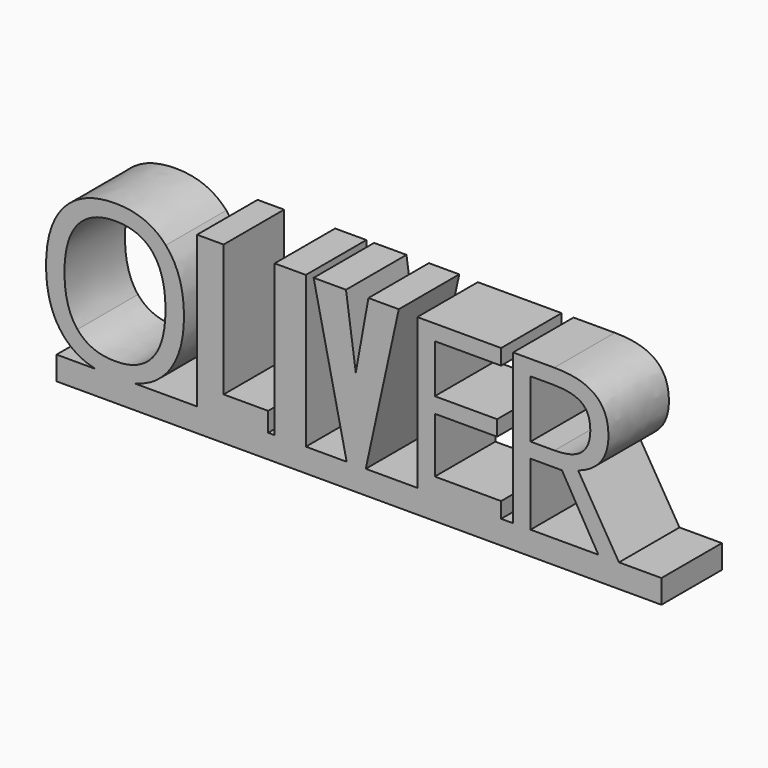
from build123d import *

# Parameters (mm, degrees)
F0_W         = 10.3234383059
F0_H         = 50
F0_TEXT_SIZE = 69.6380393088
F1_DEPTH     = 25


# Not quite as in the source:
# - Text() gives the source's letters only with a copy of the font that has no kerning and outlines rounded to 1/6400 em; it was checked with that copy


with BuildPart() as f1:
    # F0 (on Front) → F1 (new body)
    with BuildSketch(Plane.XZ):
        Polygon((-25.6522880155, 16.8570160866), (-25.6522880155, -33.1429839134), (-16.8708102065, -33.1429839134), (-2.1405949011, -33.1429839134), (-2.1405949011, -26.771583315), (-16.8708102065, -26.771583315), (-16.8708102065, 16.8570160866), align=None)
        with BuildLine():
            Line((-16.8708102065, -33.1429839134), (-25.6522880155, -33.1429839134))
            Line((-25.6522880155, -33.1429839134), (-46.4257544633, -33.1429839134))
            add(Edge.make_bspline(
                [(-46.4257544633, -33.1429839134), (-49.3466087915, -33.8265776634), (-52.7373318548, -33.8265776634)],
                knots=[0.6833950988, 0.6833950988, 0.6833950988, 1, 1, 1], degree=2))
            add(Edge.make_bspline(
                [(-52.7373318548, -33.8265776634), (-56.2343710014, -33.8265776634), (-59.2216208008, -33.1429839134)],
                knots=[0, 0, 0, 0.319412416, 0.319412416, 0.319412416], degree=2))
            Line((-59.2216208008, -33.1429839134), (-72.1091241795, -33.1429839134))
            Line((-72.1091241795, -33.1429839134), (-72.1091241795, -40.935254842))
            Line((-72.1091241795, -40.935254842), (127.8908758205, -40.935254842))
            Line((127.8908758205, -40.935254842), (127.8908758205, -33.1429839134))
            Line((127.8908758205, -33.1429839134), (113.8607155293, -33.1429839134))
            Line((113.8607155293, -33.1429839134), (107.0274829221, -33.1429839134))
            Line((107.0274829221, -33.1429839134), (84.6127390196, -33.1429839134))
            Line((84.6127390196, -33.1429839134), (78.8349579457, -33.1429839134))
            Line((78.8349579457, -33.1429839134), (74.8870150825, -33.1429839134))
            Line((74.8870150825, -33.1429839134), (47.1732516263, -33.1429839134))
            Line((47.1732516263, -33.1429839134), (30.120832633, -33.1429839134))
            Line((30.120832633, -33.1429839134), (23.8147727107, -33.1429839134))
            Line((23.8147727107, -33.1429839134), (10.3234383059, -33.1429839134))
            Line((10.3234383059, -33.1429839134), (0, -33.1429839134))
            Line((0, -33.1429839134), (-2.1405949011, -33.1429839134))
            Line((-2.1405949011, -33.1429839134), (-16.8708102065, -33.1429839134))
        make_face()
        with BuildLine():
            add(Edge.make_bspline(
                [(-46.4257544633, -33.1429839134), (-49.3466087915, -33.8265776634), (-52.7373318548, -33.8265776634)],
                knots=[0.6833950988, 0.6833950988, 0.6833950988, 1, 1, 1], degree=2))
            Line((-46.4257544633, -33.1429839134), (-59.2216208008, -33.1429839134))
            add(Edge.make_bspline(
                [(-52.7373318548, -33.8265776634), (-56.2343710014, -33.8265776634), (-59.2216208008, -33.1429839134)],
                knots=[0, 0, 0, 0.319412416, 0.319412416, 0.319412416], degree=2))
        make_face()
        with BuildLine():
            Line((-59.2216208008, -33.1429839134), (-46.4257544633, -33.1429839134))
            add(Edge.make_bspline(
                [(-36.0055610215, -27.0069162051), (-40.1210588494, -31.667439421), (-46.4257544633, -33.1429839134)],
                knots=[0, 0, 0, 0.6833950988, 0.6833950988, 0.6833950988], degree=2))
            add(Edge.make_bspline(
                [(-29.9834256048, -8.2840429412), (-29.9834256048, -20.1872547468), (-36.0055610215, -27.0069162051)],
                knots=[0, 0, 0, 1, 1, 1], degree=2))
            add(Edge.make_bspline(
                [(-35.9838596326, 10.4334049755), (-29.9834256048, 3.6517209477), (-29.9834256048, -8.2840429412)],
                knots=[0, 0, 0, 1, 1, 1], degree=2))
            add(Edge.make_bspline(
                [(-52.6722276882, 17.2150890032), (-41.9842936604, 17.2150890032), (-35.9838596326, 10.4334049755)],
                knots=[0, 0, 0, 1, 1, 1], degree=2))
            add(Edge.make_bspline(
                [(-69.6210124104, 10.5527626144), (-63.653130466, 17.2150890032), (-52.6722276882, 17.2150890032)],
                knots=[0, 0, 0, 1, 1, 1], degree=2))
            add(Edge.make_bspline(
                [(-75.5888943548, -8.2189387745), (-75.5888943548, 3.8904362255), (-69.6210124104, 10.5527626144)],
                knots=[0, 0, 0, 1, 1, 1], degree=2))
            add(Edge.make_bspline(
                [(-69.6372884521, -27.126273844), (-75.5888943548, -20.4259700245), (-75.5888943548, -8.2189387745)],
                knots=[0, 0, 0, 1, 1, 1], degree=2))
            add(Edge.make_bspline(
                [(-59.2216208008, -33.1429839134), (-65.5866993698, -31.6864174325), (-69.6372884521, -27.126273844)],
                knots=[0.319412416, 0.319412416, 0.319412416, 1, 1, 1], degree=2))
        make_face()
        with BuildLine():
            add(Edge.make_bspline(
                [(-69.4908040771, -8.2840429412), (-69.4908040771, -18.3534873856), (-65.1993544243, -23.561820719)],
                knots=[0, 0, 0, 1, 1, 1], degree=2))
            add(Edge.make_bspline(
                [(-65.1993544243, 6.8526758088), (-69.4908040771, 1.6443424755), (-69.4908040771, -8.2840429412)],
                knots=[0, 0, 0, 1, 1, 1], degree=2))
            add(Edge.make_bspline(
                [(-52.6722276882, 12.0610091421), (-60.9079047715, 12.0610091421), (-65.1993544243, 6.8526758088)],
                knots=[0, 0, 0, 1, 1, 1], degree=2))
            add(Edge.make_bspline(
                [(-40.2807346326, 6.8906532394), (-44.4691026882, 12.0610091421), (-52.6722276882, 12.0610091421)],
                knots=[0, 0, 0, 1, 1, 1], degree=2))
            add(Edge.make_bspline(
                [(-36.0923665771, -8.2840429412), (-36.0923665771, 1.7202973366), (-40.2807346326, 6.8906532394)],
                knots=[0, 0, 0, 1, 1, 1], degree=2))
            add(Edge.make_bspline(
                [(-40.2970106743, -23.5835221079), (-36.0923665771, -18.3968901634), (-36.0923665771, -8.2840429412)],
                knots=[0, 0, 0, 1, 1, 1], degree=2))
            add(Edge.make_bspline(
                [(-52.7373318548, -28.7701540523), (-44.5016547715, -28.7701540523), (-40.2970106743, -23.5835221079)],
                knots=[0, 0, 0, 1, 1, 1], degree=2))
            add(Edge.make_bspline(
                [(-65.1993544243, -23.561820719), (-60.9079047715, -28.7701540523), (-52.7373318548, -28.7701540523)],
                knots=[0, 0, 0, 1, 1, 1], degree=2))
        make_face(mode=Mode.SUBTRACT)
        with Locations((5.1617191529, -8.1429839134)):
            Rectangle(F0_W, F0_H)
        Polygon((12.8939661897, 16.8570160866), (23.8147727107, -33.1429839134), (30.120832633, -33.1429839134), (41.046527494, 16.8570160866), (31.0021188479, 16.8570160866), (26.8264431506, -6.2320148572), (23.5949363047, 16.8570160866), align=None)
        with Locations((40.3400190192, -33.1429839134)):
            Text('E', F0_TEXT_SIZE, font='Open Sans', text_align=(TextAlign.LEFT, TextAlign.BOTTOM))
        with Locations((72.0017253385, -33.1429839134)):
            Text('R', F0_TEXT_SIZE, font='Open Sans', text_align=(TextAlign.LEFT, TextAlign.BOTTOM))
    extrude(amount=F1_DEPTH)


solid = f1.part
